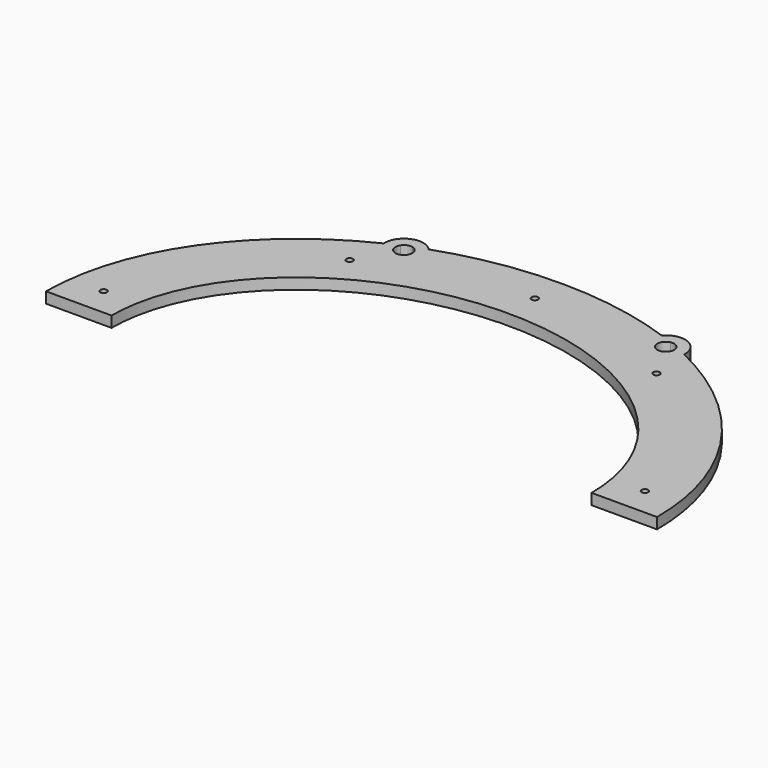
from build123d import *

# Parameters (mm, degrees)
F0_R     = 1.5
F1_DEPTH = 5


# Not quite as in the source:
# - a feature names something its author has since deleted; it is built from what else it names


with BuildPart() as f1:
    # F0 (on Top) → F1 (new body)
    with BuildSketch(Plane.XY):
        with BuildLine():
            ThreePointArc((-53.3961581093, 110.9291565406), (-63.4156131399, 113.1914108601), (-68.8598231895, 104.4811955556))
            add(Edge.make_bspline(
                [(-63.2980641383, 107.0343052721), (-66.1125104261, 105.8114732046), (-68.8598231895, 104.4811955556)],
                knots=[2.0399471573, 2.0399471573, 2.0399471573, 2.0850163371, 2.0850163371, 2.0850163371], degree=2, weights=[1, 0.9997461069, 1]))
            ThreePointArc((-63.2980641383, 107.0343052721), (-61.4906892533, 108.5767961292), (-59.1228145122, 108.7744099698))
            add(Edge.make_bspline(
                [(-53.3961581093, 110.9291565406), (-56.2875684522, 109.9066162001), (-59.1228145122, 108.7744099698)],
                knots=[1.962107852, 1.962107852, 1.962107852, 2.0067839239, 2.0067839239, 2.0067839239], degree=2, weights=[1, 0.9997505164, 1]))
        make_face()
        with BuildLine():
            add(Edge.make_bspline(
                [(-63.2980641383, 107.0343052721), (-66.1125104261, 105.8114732046), (-68.8598231895, 104.4811955556)],
                knots=[2.0399471573, 2.0399471573, 2.0399471573, 2.0850163371, 2.0850163371, 2.0850163371], degree=2, weights=[1, 0.9997461069, 1]))
            ThreePointArc((-68.8598231895, 104.4811955556), (-59.7404868081, 96.128795014), (-51.125, 105))
            ThreePointArc((-51.125, 105), (-51.7122161654, 108.1746281846), (-53.3961581093, 110.9291565406))
            add(Edge.make_bspline(
                [(-53.3961581093, 110.9291565406), (-56.2875684522, 109.9066162001), (-59.1228145122, 108.7744099698)],
                knots=[1.962107852, 1.962107852, 1.962107852, 2.0067839239, 2.0067839239, 2.0067839239], degree=2, weights=[1, 0.9997505164, 1]))
            ThreePointArc((-59.1228145122, 108.7744099698), (-56.9656369066, 107.4100343602), (-56.125, 105))
            ThreePointArc((-56.125, 105), (-61.0572668689, 101.2720230999), (-63.2980641383, 107.0343052721))
        make_face()
        with BuildLine():
            add(Edge.make_bspline(
                [(-68.8598231895, 104.4811955556), (-140, 70.0343759485), (-140, 0)],
                knots=[2.0850163371, 2.0850163371, 2.0850163371, 3.1415926536, 3.1415926536, 3.1415926536], degree=2, weights=[1, 0.863671199, 1]))
            Line((-140, 0), (-110, 0))
            add(Edge.make_bspline(
                [(110, 0), (110, 90), (0, 90), (-110, 90), (-110, 0)],
                knots=[0, 0, 0, 1.5707963268, 1.5707963268, 3.1415926536, 3.1415926536, 3.1415926536], degree=2, weights=[1, 0.7071067812, 1, 0.7071067812, 1]))
            Line((110, 0), (140, 0))
            add(Edge.make_bspline(
                [(140, 0), (140, 70.0343759485), (68.8598231895, 104.4811955556)],
                knots=[0, 0, 0, 1.0565763165, 1.0565763165, 1.0565763165], degree=2, weights=[1, 0.863671199, 1]))
            ThreePointArc((68.8598231895, 104.4811955556), (56.5843868601, 96.8085891399), (53.3961581093, 110.9291565406))
            add(Edge.make_bspline(
                [(53.3961581093, 110.9291565406), (0, 129.81257993), (-53.3961581093, 110.9291565406)],
                knots=[1.1794848016, 1.1794848016, 1.1794848016, 1.962107852, 1.962107852, 1.962107852], degree=2, weights=[1, 0.9244096378, 1]))
            ThreePointArc((-53.3961581093, 110.9291565406), (-51.7122161654, 108.1746281846), (-51.125, 105))
            ThreePointArc((-51.125, 105), (-59.7404868081, 96.128795014), (-68.8598231895, 104.4811955556))
        make_face()
        with Locations((-124.0382502632, 13)):
            Circle(F0_R, mode=Mode.SUBTRACT)
        with Locations((-70.333152659, 86.8019097296)):
            Circle(F0_R, mode=Mode.SUBTRACT)
        with Locations((124.0382502632, 13)):
            Circle(F0_R, mode=Mode.SUBTRACT)
        with Locations((0, 105)):
            Circle(F0_R, mode=Mode.SUBTRACT)
        with Locations((70.333152659, 86.8019097296)):
            Circle(F0_R, mode=Mode.SUBTRACT)
        with BuildLine():
            add(Edge.make_bspline(
                [(68.8598231895, 104.4811955556), (66.1125104261, 105.8114732046), (63.2980641383, 107.0343052721)],
                knots=[1.0565763165, 1.0565763165, 1.0565763165, 1.1016454963, 1.1016454963, 1.1016454963], degree=2, weights=[1, 0.9997461069, 1]))
            ThreePointArc((68.8598231895, 104.4811955556), (68.871204986, 104.7404868081), (68.875, 105))
            ThreePointArc((68.875, 105), (63.1746281846, 113.2877838346), (53.3961581093, 110.9291565406))
            add(Edge.make_bspline(
                [(59.1228145122, 108.7744099698), (56.2875684522, 109.9066162001), (53.3961581093, 110.9291565406)],
                knots=[1.1348087297, 1.1348087297, 1.1348087297, 1.1794848016, 1.1794848016, 1.1794848016], degree=2, weights=[1, 0.9997505164, 1]))
            ThreePointArc((59.1228145122, 108.7744099698), (61.4906892533, 108.5767961292), (63.2980641383, 107.0343052721))
        make_face()
        with BuildLine():
            ThreePointArc((53.3961581093, 110.9291565406), (56.5843868601, 96.8085891399), (68.8598231895, 104.4811955556))
            add(Edge.make_bspline(
                [(68.8598231895, 104.4811955556), (66.1125104261, 105.8114732046), (63.2980641383, 107.0343052721)],
                knots=[1.0565763165, 1.0565763165, 1.0565763165, 1.1016454963, 1.1016454963, 1.1016454963], degree=2, weights=[1, 0.9997461069, 1]))
            ThreePointArc((63.2980641383, 107.0343052721), (63.7279769001, 106.0572668689), (63.875, 105))
            ThreePointArc((63.875, 105), (57.5899656398, 101.9656369066), (59.1228145122, 108.7744099698))
            add(Edge.make_bspline(
                [(59.1228145122, 108.7744099698), (56.2875684522, 109.9066162001), (53.3961581093, 110.9291565406)],
                knots=[1.1348087297, 1.1348087297, 1.1348087297, 1.1794848016, 1.1794848016, 1.1794848016], degree=2, weights=[1, 0.9997505164, 1]))
        make_face()
    extrude(amount=F1_DEPTH)


solid = f1.part
